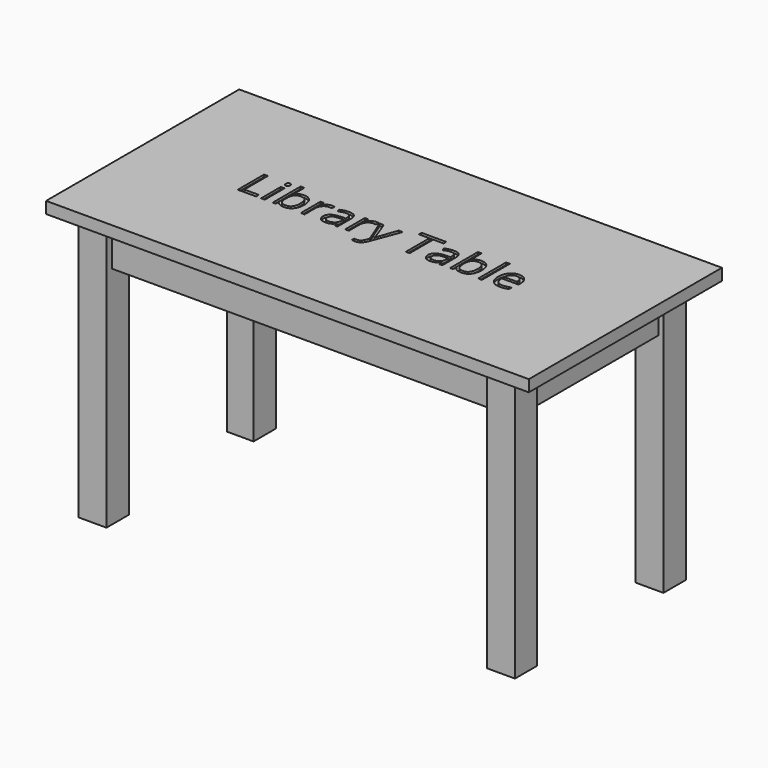
from build123d import *

# Parameters (mm, degrees)
F0_W         = 76.2
F0_H         = 76.2
F1_DEPTH     = 730.25
F0_H_2       = 76.3438940048
F0_W_2       = 72.3258499056
F2_W         = 1158.7507165968
F2_H         = 548.3160167933
F3_DEPTH     = 114.3
F4_W         = 1320.8
F4_H         = 660.4
F5_DEPTH     = 31.75
F6_TEXT_SIZE = 125.7340113322
F7_DEPTH     = 6.35


# Not quite as in the source:
# - a length typed as a fraction of an inch, garbled in the dataset ("3 / 203.2 mm" for 3/8 in), is restored
# - Text() gives the source's letters only with a copy of the font that has no kerning and outlines rounded to 1/6400 em; it was checked with that copy


with BuildPart() as f1:
    # F0 (on Top) → F1 (new body)
    with BuildSketch(Plane.XY):
        with Locations((38.1, 38.1)):
            Rectangle(F0_W, F0_H)
    extrude(amount=F1_DEPTH)


with BuildPart() as f1b:
    # F0 (on Top) → F1, piece 2 (new body)
    with BuildSketch(Plane.XY):
        with Locations((1155.7, 38.1)):
            Rectangle(F0_W, F0_H)
    extrude(amount=F1_DEPTH)


with BuildPart() as f1c:
    # F0 (on Top) → F1, piece 3 (new body)
    with BuildSketch(Plane.XY):
        with Locations((1155.7, 546.0280529976)):
            Rectangle(F0_W, F0_H_2)
    extrude(amount=F1_DEPTH)


with BuildPart() as f1d:
    # F0 (on Top) → F1, piece 4 (new body)
    with BuildSketch(Plane.XY):
        with Locations((36.1629249528, 546.0280529976)):
            Rectangle(F0_W_2, F0_H_2)
    extrude(amount=F1_DEPTH)


with BuildPart() as f3:
    # F2 (on face) → F3 (new body)
    with BuildSketch(Plane.XY.offset(730.25)):
        with Locations((600.8832734078, 293.4529706836)):
            Rectangle(F2_W, F2_H)
    extrude(amount=-F3_DEPTH)

    # F4 (on face) → F5 (join)
    with BuildSketch(Plane.XY.offset(730.25)):
        with Locations((605.4751439661, 287.5400213525)):
            Rectangle(F4_W, F4_H)
    extrude(amount=F5_DEPTH)

    # F6 (on face) → F7 (cut)
    with BuildSketch(Plane.XY.offset(762)):
        with Locations((220.3024029732, 253.4461915493)):
            Text('Library Table', F6_TEXT_SIZE, font='Open Sans', text_align=(TextAlign.LEFT, TextAlign.BOTTOM))
    extrude(amount=-F7_DEPTH, mode=Mode.SUBTRACT)


solid = Compound([f1.part, f1b.part, f1c.part, f1d.part, f3.part])
